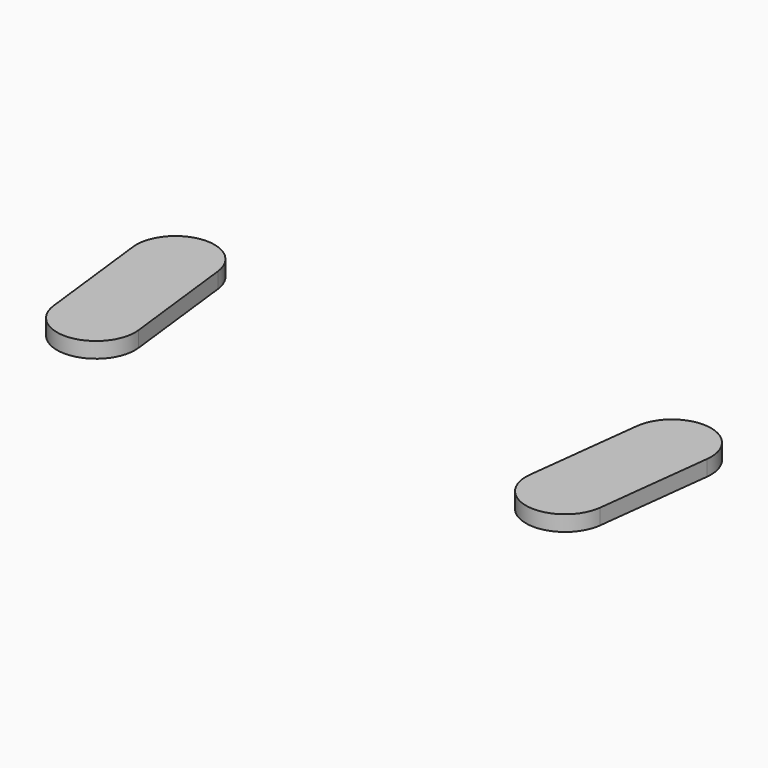
from build123d import *

# Parameters (mm, degrees)
F1_DEPTH = 2


# Not quite as in the source:
# - the program builds the solid bodies; features that only make, move or delete a surface that nothing else refers to are left out


with BuildPart() as f1:
    # F0 (on Top) → F1 (new body)
    with BuildSketch(Plane.XY):
        with BuildLine():
            Line((-36.7307308238, 32.6093674274), (-26.8, 33.7843505361))
            ThreePointArc((-26.8, 33.7843505361), (-32.3528569662, 38.1622243937), (-36.7307308238, 32.6093674274))
        make_face()
        Polygon((-25.037525337, 18.8882543005), (-26.8, 33.7843505361), (-36.7307308238, 32.6093674274), (-34.9682561607, 17.7132711918), align=None)
        with BuildLine():
            ThreePointArc((-34.9682561607, 17.7132711918), (-29.4153991945, 13.3353973342), (-25.037525337, 18.8882543005))
            Line((-25.037525337, 18.8882543005), (-34.9682561607, 17.7132711918))
        make_face()
    extrude(amount=F1_DEPTH)


with BuildPart() as f1b:
    # F0 (on Top) → F1, piece 2 (new body)
    with BuildSketch(Plane.XY):
        with BuildLine():
            Line((34.9682561607, 17.7132711918), (25.037525337, 18.8882543005))
            ThreePointArc((25.037525337, 18.8882543005), (29.4153991945, 13.3353973342), (34.9682561607, 17.7132711918))
        make_face()
        Polygon((36.7307308238, 32.6093674274), (26.8, 33.7843505361), (25.037525337, 18.8882543005), (34.9682561607, 17.7132711918), align=None)
        with BuildLine():
            ThreePointArc((36.7307308238, 32.6093674274), (32.3528569662, 38.1622243937), (26.8, 33.7843505361))
            Line((26.8, 33.7843505361), (36.7307308238, 32.6093674274))
        make_face()
    extrude(amount=F1_DEPTH)


solid = Compound([f1.part, f1b.part])
